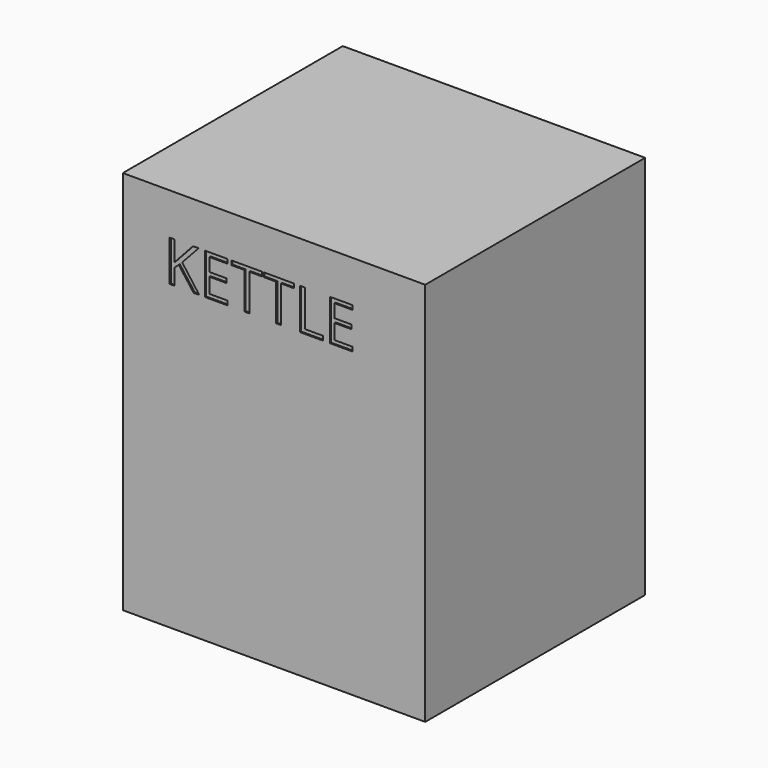
from build123d import *

# Parameters (mm, degrees)
F0_W         = 220
F0_H         = 200
F1_DEPTH     = 280
F2_TEXT_SIZE = 41.6666666667
F3_DEPTH     = 1


# Not quite as in the source:
# - Text() gives the source's letters only with a copy of the font that has no kerning and outlines rounded to 1/6400 em; it was checked with that copy


with BuildPart() as f1:
    # F0 (on Top) → F1 (new body)
    with BuildSketch(Plane.XY):
        Rectangle(F0_W, F0_H)
    extrude(amount=F1_DEPTH)

    # F2 (on face) → F3 (cut)
    with BuildSketch(Plane.XZ.offset(100)):
        with Locations((-80, 220)):
            Text('KETTLE', F2_TEXT_SIZE, font='Open Sans', text_align=(TextAlign.LEFT, TextAlign.BOTTOM))
    extrude(amount=-F3_DEPTH, mode=Mode.SUBTRACT)


solid = f1.part
